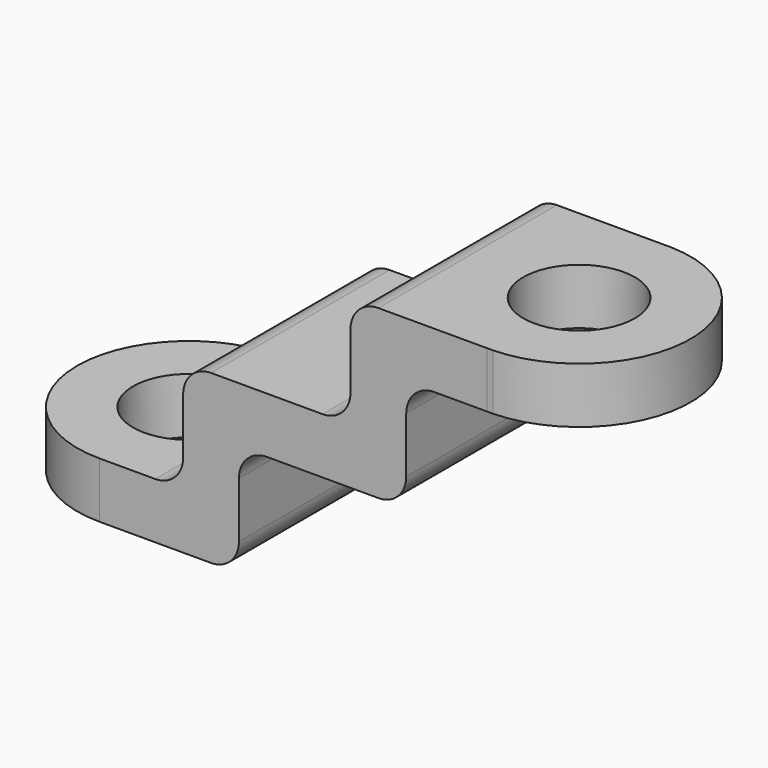
from build123d import *

# Parameters (mm, degrees)
F0_R     = 100
F1_DEPTH = 500
F3_DEPTH = 300


# Not quite as in the source:
# - ends of sketch curves that miss each other by under 0.0002 mm in the source are joined


with BuildPart() as f1:
    # F0 (on Top) → F1 (new body)
    with BuildSketch(Plane.XY):
        with BuildLine():
            Line((344.892811266, 199.9347809243), (-349.9812287722, 199.9999991191))
            ThreePointArc((-349.9812287722, 199.9999991191), (-550, 0), (-349.9812287722, -199.9999991191))
            Line((-349.9812287722, -199.9999991191), (344.892811266, -199.9347809243))
            Line((344.892811266, -199.9347809243), (355.1449138709, -199.9338187015))
            ThreePointArc((355.1449138709, -199.9338187015), (550, 9.74749e-05), (355.1447188571, 199.9338187198))
            Line((355.1447188571, 199.9338187198), (344.892811266, 199.9347809243))
        make_face()
        with Locations((-350, 0)):
            Circle(F0_R, mode=Mode.SUBTRACT)
        with Locations((350, 0)):
            Circle(F0_R, mode=Mode.SUBTRACT)
    extrude(amount=F1_DEPTH)


with BuildPart() as f3:
    # F2 (on Front) → F3 (new body, symmetric)
    with BuildSketch(Plane.XZ):
        with BuildLine():
            Line((-550, 100), (-550, 0))
            Line((-550, 0), (-150, 0))
            ThreePointArc((-150, 0), (-114.6446609407, 14.6446609407), (-100, 50))
            Line((-100, 50), (-100, 150))
            ThreePointArc((-100, 150), (-85.3553390593, 185.3553390593), (-50, 200))
            Line((-50, 200), (150, 200))
            ThreePointArc((150, 200), (185.3553390593, 214.6446609407), (200, 250))
            Line((200, 250), (200, 350))
            ThreePointArc((200, 350), (214.6446609407, 385.3553390593), (250, 400))
            Line((250, 400), (550, 400))
            Line((550, 400), (550, 500))
            Line((550, 500), (150, 500))
            ThreePointArc((150, 500), (114.6446609407, 485.3553390593), (100, 450))
            Line((100, 450), (100, 350))
            ThreePointArc((100, 350), (85.3553390593, 314.6446609407), (50, 300))
            Line((50, 300), (-150, 300))
            ThreePointArc((-150, 300), (-185.3553390593, 285.3553390593), (-200, 250))
            Line((-200, 250), (-200, 150))
            ThreePointArc((-200, 150), (-214.6446609407, 114.6446609407), (-250, 100))
            Line((-250, 100), (-550, 100))
        make_face()
    extrude(amount=F3_DEPTH, both=True)


with BuildPart() as f1_1:
    add(f1.part)

    # F4: intersect F3
    add(f3.part, mode=Mode.INTERSECT)


solid = f1_1.part
